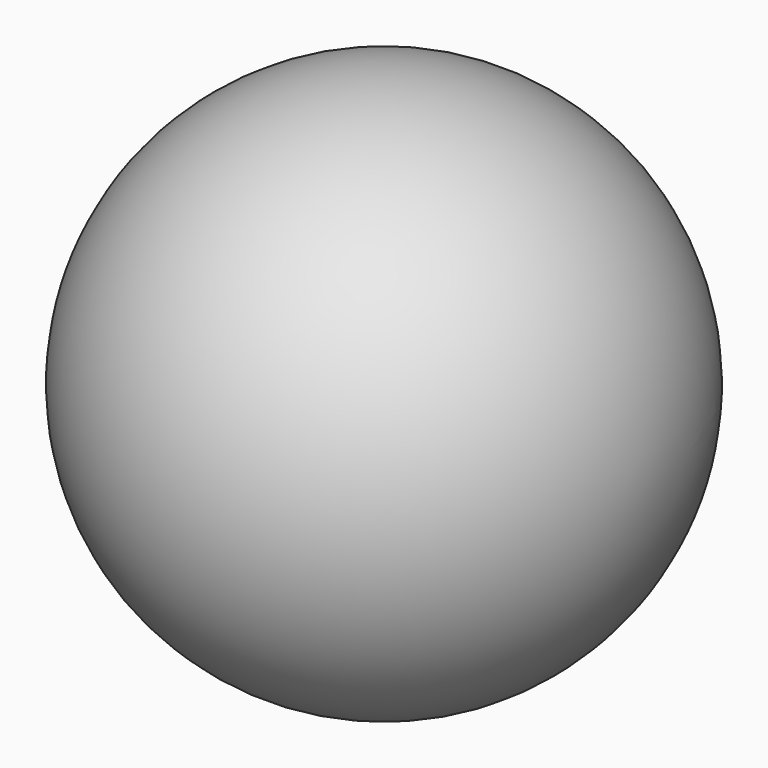
from build123d import *


# Not quite as in the source:
# - a feature of the source that left no trace in its solid (it failed there, or was rolled back) is left out


with BuildPart() as f2:
    # F0 (on Top) → F2 (revolve)
    with BuildSketch(Plane.XY):
        with BuildLine():
            Line((23.8125, 0), (25.4, 0))
            ThreePointArc((25.4, 0), (0, 25.4), (-25.4, 0))
            Line((-25.4, 0), (-23.8125, 0))
            ThreePointArc((-23.8125, 0), (0, 23.8125), (23.8125, 0))
        make_face()
    revolve(axis=Axis((0, 0, 0), (1, 0, 0)))


solid = f2.part
